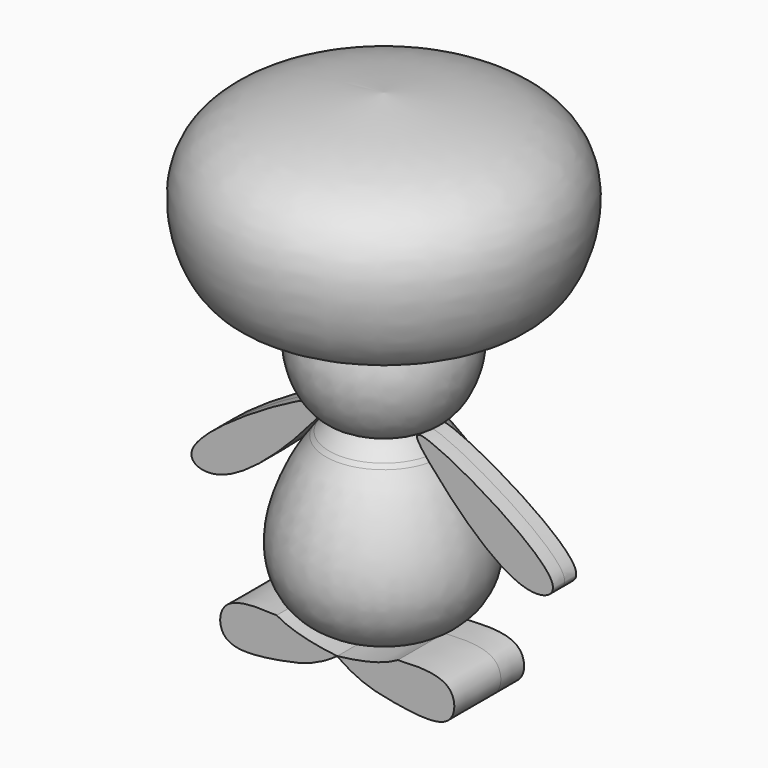
from build123d import *

# Parameters (mm, degrees)
F2_DEPTH = 3.175
F3_DEPTH = 12.7
F4_DEPTH = 6.35


with BuildPart() as f1:
    # F0 (on Front) → F1 (revolve)
    with BuildSketch(Plane.XZ):
        with BuildLine():
            Line((0, 40.5440760271), (0, 71.9247758389))
            add(Edge.make_bspline(
                [(0, 71.9247758389), (-10.5854645625, 70.8659542485), (-28.8822806187, 69.0357970776), (-39.9716556363, 54.991269554), (-32.0733651409, 29.2208619873), (-17.841770712, 34.9733702393), (-12.2893932233, 36.4083050153)],
                knots=[0, 0, 0, 0, 0.2498962885, 0.4319419707, 0.6419249767, 0.8356777921, 0.8356777921, 0.8356777921, 0.8356777921], degree=3))
            add(Edge.make_bspline(
                [(0, 40.5440760271), (-4.5284186079, 40.0266843128), (-9.0312162462, 39.2304703796), (-12.2893932233, 36.4083050153)],
                knots=[0, 0, 0, 0, 0.2308023195, 0.2308023195, 0.2308023195, 0.2308023195], degree=3))
        make_face()
        with BuildLine():
            Line((0, 38.1521359086), (0, 40.5440760271))
            add(Edge.make_bspline(
                [(0, 40.5440760271), (-4.5284186079, 40.0266843128), (-9.0312162462, 39.2304703796), (-12.2893932233, 36.4083050153)],
                knots=[0, 0, 0, 0, 0.2308023195, 0.2308023195, 0.2308023195, 0.2308023195], degree=3))
            add(Edge.make_bspline(
                [(-12.2893932233, 36.4083050153), (-7.5804091174, 37.6252764959), (-3.7902045587, 37.8887062023), (0, 38.1521359086)],
                knots=[0.8356777921, 0.8356777921, 0.8356777921, 0.8356777921, 1, 1, 1, 1], degree=3))
        make_face()
        with BuildLine():
            add(Edge.make_bspline(
                [(-12.2893932233, 36.4083050153), (-7.5804091174, 37.6252764959), (-3.7902045587, 37.8887062023), (0, 38.1521359086)],
                knots=[0.8356777921, 0.8356777921, 0.8356777921, 0.8356777921, 1, 1, 1, 1], degree=3))
            add(Edge.make_bspline(
                [(-12.2893932233, 36.4083050153), (-15.7284594552, 33.4294571278), (-19.7950616175, 23.0549580863), (-13.8903816598, 12.283135182), (-10.3272052615, 10.8123944002)],
                knots=[0.2308023195, 0.2308023195, 0.2308023195, 0.2308023195, 0.4744184485, 0.713498165, 0.713498165, 0.713498165, 0.713498165], degree=3))
            add(Edge.make_bspline(
                [(-10.3272052615, 10.8123944002), (-10.0725579486, 10.8090009422), (-9.9059347314, 10.7453373429), (-9.8162787914, 10.6283200932)],
                knots=[0.8548334172, 0.8548334172, 0.8548334172, 0.8548334172, 0.8798658908, 0.8798658908, 0.8798658908, 0.8798658908], degree=3))
            add(Edge.make_bspline(
                [(-9.8162787914, 10.6283200932), (-9.1137535972, 10.4101545267), (-8.3931801359, 10.322881828), (-7.6793552666, 10.3051986154)],
                knots=[0.7248371265, 0.7248371265, 0.7248371265, 0.7248371265, 0.7712842823, 0.7712842823, 0.7712842823, 0.7712842823], degree=3))
            add(Edge.make_bspline(
                [(-3.1846784663, 10.5425213196), (-4.6581488019, 10.9051649254), (-6.1325150121, 10.9671798034), (-7.6793552671, 10.3051986181)],
                knots=[0.0710045794, 0.0710045794, 0.0710045794, 0.0710045794, 0.1703333243, 0.1703333243, 0.1703333243, 0.1703333243], degree=3))
            add(Edge.make_bspline(
                [(-3.1846784663, 10.5425213196), (-3.0362223015, 10.5371579355), (-1.6218651964, 10.4344784463), (-0.6951761314, 9.7262982289), (0, 9.4586049693)],
                knots=[0.8774986759, 0.8774986759, 0.8774986759, 0.8774986759, 0.8899612006, 1, 1, 1, 1], degree=3))
            Line((0, 9.4586049693), (0, 38.1521359086))
        make_face()
    revolve(axis=Axis((0, 0, 0.5056373775), (0, 0, -1)))


with BuildPart() as f1b:
    # F0 (on Front) → F1, piece 2 (revolve)
    with BuildSketch(Plane.XZ):
        with BuildLine():
            add(Edge.make_bspline(
                [(0, 9.4586049693), (1.0785327456, 9.8704319859), (2.131376709, 10.2832876329), (3.1846784663, 10.5425213196)],
                knots=[0, 0, 0, 0, 0.0710045794, 0.0710045794, 0.0710045794, 0.0710045794], degree=3))
            Line((0, 9.4586049693), (0, 0))
            Line((0, 0), (0, -31.173305586))
            add(Edge.make_bspline(
                [(13.22216002, -27.6354453357), (10.0983043363, -29.4406761674), (5.8726727159, -30.4915417833), (0, -31.173305586)],
                knots=[0.8141867643, 0.8141867643, 0.8141867643, 0.8141867643, 1, 1, 1, 1], degree=3))
            add(Edge.make_bspline(
                [(12.621386915, 6.0216014374), (16.0083791906, 1.743010511), (22.5080544597, -12.133560287), (19.2333086543, -23.0820491065), (14.6028300587, -26.8375761719), (13.22216002, -27.6354453357)],
                knots=[0.2734670882, 0.2734670882, 0.2734670882, 0.2734670882, 0.4878925442, 0.732061726, 0.8141867643, 0.8141867643, 0.8141867643, 0.8141867643], degree=3))
            add(Edge.make_bspline(
                [(11.8949395762, 6.8987859434), (12.1253138051, 6.6158984029), (12.3684349547, 6.322895519), (12.621386915, 6.0216014374)],
                knots=[0.9839467979, 0.9839467979, 0.9839467979, 0.9839467979, 1, 1, 1, 1], degree=3))
            add(Edge.make_bspline(
                [(7.6793552671, 10.3051986181), (7.8497440907, 10.2322795206), (9.2257027917, 9.5758758934), (10.664594848, 8.3159473687), (11.8949395762, 6.8987859434)],
                knots=[0.1703333243, 0.1703333243, 0.1703333243, 0.1703333243, 0.1812746661, 0.2582354256, 0.2582354256, 0.2582354256, 0.2582354256], degree=3))
            add(Edge.make_bspline(
                [(7.6793552666, 10.3051986154), (6.0469953416, 10.2647610112), (4.4499262301, 10.5882318478), (3.1846784663, 10.5425213196)],
                knots=[0.7712842823, 0.7712842823, 0.7712842823, 0.7712842823, 0.8774986759, 0.8774986759, 0.8774986759, 0.8774986759], degree=3))
        make_face()
    revolve(axis=Axis((0, 0, 0.5056373775), (0, 0, -1)))


with BuildPart() as f2:
    # F0 (on Front) → F2 (new body, symmetric)
    with BuildSketch(Plane.XZ):
        with BuildLine():
            add(Edge.make_bspline(
                [(-10.3272052615, 10.8123944002), (-10.1582125886, 10.7426407905), (-9.9877835061, 10.6815799955), (-9.8162787914, 10.6283200932)],
                knots=[0.713498165, 0.713498165, 0.713498165, 0.713498165, 0.7248371265, 0.7248371265, 0.7248371265, 0.7248371265], degree=3))
            add(Edge.make_bspline(
                [(-12.621386915, 6.0216014374), (-17.8399461837, -0.1942864324), (-31.5853075666, -14.4396466007), (-46.6922995721, -7.7363055156), (-14.0981138501, 10.862645941), (-10.3272052615, 10.8123944002)],
                knots=[0, 0, 0, 0, 0.3311877351, 0.4841435846, 0.8548334172, 0.8548334172, 0.8548334172, 0.8548334172], degree=3))
            add(Edge.make_bspline(
                [(-11.8949395762, 6.8987859434), (-12.1384428364, 6.6183089198), (-12.3807927025, 6.3255301539), (-12.621386915, 6.0216014374)],
                knots=[0.2582354256, 0.2582354256, 0.2582354256, 0.2582354256, 0.2734670882, 0.2734670882, 0.2734670882, 0.2734670882], degree=3))
            add(Edge.make_bspline(
                [(-9.8162787914, 10.6283200932), (-9.4435041431, 10.1417816202), (-10.4013086806, 8.7328867997), (-11.8949395762, 6.8987859434)],
                knots=[0.8798658908, 0.8798658908, 0.8798658908, 0.8798658908, 0.9839467979, 0.9839467979, 0.9839467979, 0.9839467979], degree=3))
        make_face()
    extrude(amount=F2_DEPTH, both=True)


with BuildPart() as f2b:
    # F0 (on Front) → F2, piece 2 (new body, symmetric)
    with BuildSketch(Plane.XZ):
        with BuildLine():
            add(Edge.make_bspline(
                [(12.621386915, 6.0216014374), (17.8399461837, -0.1942864324), (31.5853075666, -14.4396466007), (46.6922995721, -7.7363055156), (14.0981138501, 10.862645941), (10.3272052615, 10.8123944002)],
                knots=[0, 0, 0, 0, 0.3311877351, 0.4841435846, 0.8548334172, 0.8548334172, 0.8548334172, 0.8548334172], degree=3))
            add(Edge.make_bspline(
                [(10.3272052615, 10.8123944002), (10.1582125886, 10.7426407905), (9.9877835061, 10.6815799955), (9.8162787914, 10.6283200932)],
                knots=[0.713498165, 0.713498165, 0.713498165, 0.713498165, 0.7248371265, 0.7248371265, 0.7248371265, 0.7248371265], degree=3))
            add(Edge.make_bspline(
                [(9.8162787914, 10.6283200932), (9.4435041431, 10.1417816202), (10.4013086806, 8.7328867997), (11.8949395762, 6.8987859434)],
                knots=[0.8798658908, 0.8798658908, 0.8798658908, 0.8798658908, 0.9839467979, 0.9839467979, 0.9839467979, 0.9839467979], degree=3))
            add(Edge.make_bspline(
                [(11.8949395762, 6.8987859434), (12.1384428364, 6.6183089198), (12.3807927025, 6.3255301539), (12.621386915, 6.0216014374)],
                knots=[0.2582354256, 0.2582354256, 0.2582354256, 0.2582354256, 0.2734670882, 0.2734670882, 0.2734670882, 0.2734670882], degree=3))
        make_face()
    extrude(amount=F2_DEPTH, both=True)


with BuildPart() as f3:
    # F0 (on Front) → F3 (new body)
    with BuildSketch(Plane.XZ):
        with BuildLine():
            add(Edge.make_bspline(
                [(13.22216002, -27.6354453357), (17.3132413575, -27.4060696494), (25.9248047573, -27.1058110564), (25.9056330976, -37.9555936987), (11.9017516816, -36.1506097667), (4.7044344075, -34.5888761575), (0, -31.173305586)],
                knots=[0, 0, 0, 0, 0.2603616875, 0.4500846903, 0.7089889209, 1, 1, 1, 1], degree=3))
            add(Edge.make_bspline(
                [(13.22216002, -27.6354453357), (10.0983043363, -29.4406761674), (5.8726727159, -30.4915417833), (0, -31.173305586)],
                knots=[0.8141867643, 0.8141867643, 0.8141867643, 0.8141867643, 1, 1, 1, 1], degree=3))
        make_face()
    extrude(amount=F3_DEPTH)


with BuildPart() as f3b:
    # F0 (on Front) → F3, piece 2 (new body)
    with BuildSketch(Plane.XZ):
        with BuildLine():
            add(Edge.make_bspline(
                [(-13.22216002, -27.6354453357), (-10.0983043363, -29.4406761674), (-5.8726727159, -30.4915417833), (0, -31.173305586)],
                knots=[0.8141867643, 0.8141867643, 0.8141867643, 0.8141867643, 1, 1, 1, 1], degree=3))
            add(Edge.make_bspline(
                [(-13.22216002, -27.6354453357), (-17.3132413575, -27.4060696494), (-25.9248047573, -27.1058110564), (-25.9056330976, -37.9555936987), (-11.9017516816, -36.1506097667), (-4.7044344075, -34.5888761575), (0, -31.173305586)],
                knots=[0, 0, 0, 0, 0.2603616875, 0.4500846903, 0.7089889209, 1, 1, 1, 1], degree=3))
        make_face()
    extrude(amount=F3_DEPTH)


with BuildPart() as f4:
    # F0 (on Front) → F4 (new body)
    with BuildSketch(Plane.XZ):
        with BuildLine():
            add(Edge.make_bspline(
                [(13.22216002, -27.6354453357), (17.3132413575, -27.4060696494), (25.9248047573, -27.1058110564), (25.9056330976, -37.9555936987), (11.9017516816, -36.1506097667), (4.7044344075, -34.5888761575), (0, -31.173305586)],
                knots=[0, 0, 0, 0, 0.2603616875, 0.4500846903, 0.7089889209, 1, 1, 1, 1], degree=3))
            add(Edge.make_bspline(
                [(13.22216002, -27.6354453357), (10.0983043363, -29.4406761674), (5.8726727159, -30.4915417833), (0, -31.173305586)],
                knots=[0.8141867643, 0.8141867643, 0.8141867643, 0.8141867643, 1, 1, 1, 1], degree=3))
        make_face()
    extrude(amount=-F4_DEPTH)


with BuildPart() as f4b:
    # F0 (on Front) → F4, piece 2 (new body)
    with BuildSketch(Plane.XZ):
        with BuildLine():
            add(Edge.make_bspline(
                [(-13.22216002, -27.6354453357), (-10.0983043363, -29.4406761674), (-5.8726727159, -30.4915417833), (0, -31.173305586)],
                knots=[0.8141867643, 0.8141867643, 0.8141867643, 0.8141867643, 1, 1, 1, 1], degree=3))
            add(Edge.make_bspline(
                [(-13.22216002, -27.6354453357), (-17.3132413575, -27.4060696494), (-25.9248047573, -27.1058110564), (-25.9056330976, -37.9555936987), (-11.9017516816, -36.1506097667), (-4.7044344075, -34.5888761575), (0, -31.173305586)],
                knots=[0, 0, 0, 0, 0.2603616875, 0.4500846903, 0.7089889209, 1, 1, 1, 1], degree=3))
        make_face()
    extrude(amount=-F4_DEPTH)


solid = Compound([f1.part, f1b.part, f2.part, f2b.part, f3.part, f3b.part, f4.part, f4b.part])
